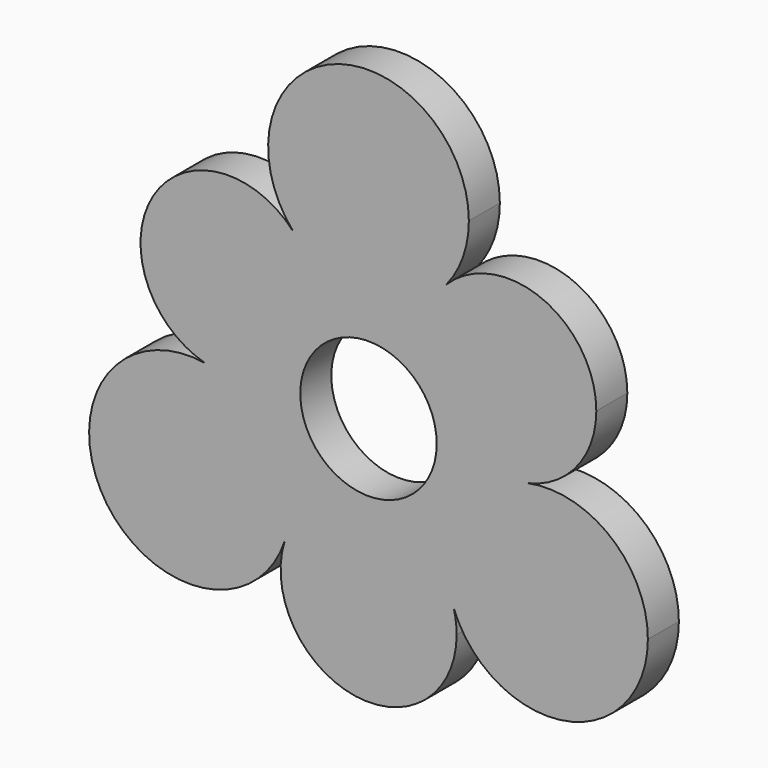
from build123d import *

# Parameters (mm, degrees)
F0_R     = 11.176
F1_DEPTH = 6.35


with BuildPart() as f1:
    # F0 (on Front) → F1 (new body)
    with BuildSketch(Plane.XZ):
        with BuildLine():
            ThreePointArc((12.7517006508, 23.4892014836), (15.490274076, 28.359134381), (16.4396849361, 33.8650085032))
            ThreePointArc((16.4396849361, 33.8650085032), (-5.7959286408, 49.2491058764), (-12.3528926478, 23.0174611293))
            ThreePointArc((-12.3528926478, 23.0174611293), (-12.2109180853, 22.8621908621), (-12.0712241226, 22.7048656287))
            ThreePointArc((-12.0712241226, 22.7048656287), (-0.3017671927, 17.4280934228), (11.6534468913, 22.2693016964))
            ThreePointArc((11.6534468913, 22.2693016964), (12.1852012792, 22.8948917308), (12.7517006508, 23.4892014836))
        make_face()
        with BuildLine():
            ThreePointArc((-12.0712241226, 22.7048656287), (-12.2109180853, 22.8621908621), (-12.3528926478, 23.0174611293))
            ThreePointArc((-12.3528926478, 23.0174611293), (-12.2130585437, 22.8602621723), (-12.0712241226, 22.7048656287))
        make_face()
        with BuildLine():
            ThreePointArc((-12.0712241226, 22.7048656287), (-12.2130585437, 22.8602621723), (-12.3528926478, 23.0174611293))
            ThreePointArc((-12.3528926478, 23.0174611293), (-35.2568762282, 20.6796890684), (-26.7180955248, -0.7013040367))
            ThreePointArc((-26.7180955248, -0.7013040367), (-25.9110393194, -0.8518354275), (-25.1125044392, -1.0424697987))
            ThreePointArc((-25.1125044392, -1.0424697987), (-13.5329586121, 2.2669935247), (-8.5036933239, 13.2097957122))
            ThreePointArc((-8.5036933239, 13.2097957122), (-9.4250093039, 18.2813740839), (-12.0712241226, 22.7048656287))
        make_face()
        with BuildLine():
            ThreePointArc((37.321032921, 13.2471223209), (28.4497702153, 26.5564449349), (12.7517006508, 23.4892014836))
            ThreePointArc((12.7517006508, 23.4892014836), (12.2178085396, 22.8655360028), (11.6534468913, 22.2693016964))
            ThreePointArc((11.6534468913, 22.2693016964), (10.5710761807, 5.7719047545), (25.6986024853, -0.8984460694))
            ThreePointArc((25.6986024853, -0.8984460694), (25.9040970502, -0.8533121295), (26.1101523925, -0.8108117214))
            ThreePointArc((26.1101523925, -0.8108117214), (34.1751435518, 4.2567197748), (37.321032921, 13.2471223209))
        make_face()
        with BuildLine():
            ThreePointArc((11.6534468913, 22.2693016964), (12.2178085396, 22.8655360028), (12.7517006508, 23.4892014836))
            ThreePointArc((12.7517006508, 23.4892014836), (12.1852012792, 22.8948917308), (11.6534468913, 22.2693016964))
        make_face()
        with BuildLine():
            ThreePointArc((-25.1125044392, -1.0424697987), (-25.9201584954, -0.8947520073), (-26.7180955248, -0.7013040367))
            ThreePointArc((-26.7180955248, -0.7013040367), (-43.4081977491, -25.41837957), (-13.7572597447, -22.2066494078))
            ThreePointArc((-13.7572597447, -22.2066494078), (-13.6937790301, -22.0060606965), (-13.6273783627, -21.8064195594))
            ThreePointArc((-13.6273783627, -21.8064195594), (-13.0740993856, -19.3973230871), (-12.8882727271, -16.9325042516))
            ThreePointArc((-12.8882727271, -16.9325042516), (-16.2979161501, -6.9084701851), (-25.1125044392, -1.0424697987))
        make_face()
        with BuildLine():
            ThreePointArc((-25.1125044392, -1.0424697987), (-25.9110393194, -0.8518354275), (-26.7180955248, -0.7013040367))
            ThreePointArc((-26.7180955248, -0.7013040367), (-25.9201584954, -0.8947520073), (-25.1125044392, -1.0424697987))
        make_face()
        with BuildLine():
            ThreePointArc((-13.6273783627, -21.8064195594), (-13.6937790301, -22.0060606965), (-13.7572597447, -22.2066494078))
            ThreePointArc((-13.7572597447, -22.2066494078), (-13.6910385066, -22.0069500429), (-13.6273783627, -21.8064195594))
        make_face()
        with BuildLine():
            ThreePointArc((-13.6273783627, -21.8064195594), (-13.6910385066, -22.0069500429), (-13.7572597447, -22.2066494078))
            ThreePointArc((-13.7572597447, -22.2066494078), (-2.127588621, -40.7153049273), (14.44099559, -26.4569180331))
            ThreePointArc((14.44099559, -26.4569180331), (14.3218531968, -24.6071235917), (13.966394874, -22.7878974469))
            ThreePointArc((13.966394874, -22.7878974469), (13.6932307798, -22.0137005753), (13.459057548, -21.2268318977))
            ThreePointArc((13.459057548, -21.2268318977), (-0.2869219447, -12.0407728951), (-13.6273783627, -21.8064195594))
        make_face()
        with BuildLine():
            ThreePointArc((26.1101523925, -0.8108117214), (25.9046971154, -0.8561301656), (25.6986024853, -0.8984460694))
            ThreePointArc((25.6986024853, -0.8984460694), (15.24405524, -8.4527086566), (13.459057548, -21.2268318977))
            ThreePointArc((13.459057548, -21.2268318977), (13.7349572161, -22.0001397234), (13.966394874, -22.7878974469))
            ThreePointArc((13.966394874, -22.7878974469), (32.3048678413, -33.100412174), (45.7676425992, -16.9325042516))
            ThreePointArc((45.7676425992, -16.9325042516), (39.7530124822, -4.2210341235), (26.1101523925, -0.8108117214))
        make_face()
        with BuildLine():
            ThreePointArc((26.1101523925, -0.8108117214), (25.9040970502, -0.8533121295), (25.6986024853, -0.8984460694))
            ThreePointArc((25.6986024853, -0.8984460694), (25.9046971154, -0.8561301656), (26.1101523925, -0.8108117214))
        make_face()
        with BuildLine():
            ThreePointArc((13.966394874, -22.7878974469), (13.7349572161, -22.0001397234), (13.459057548, -21.2268318977))
            ThreePointArc((13.459057548, -21.2268318977), (13.6932307798, -22.0137005753), (13.966394874, -22.7878974469))
        make_face()
        with BuildLine():
            ThreePointArc((11.6534468913, 22.2693016964), (-0.3017671927, 17.4280934228), (-12.0712241226, 22.7048656287))
            ThreePointArc((-12.0712241226, 22.7048656287), (-9.4250093039, 18.2813740839), (-8.5036933239, 13.2097957122))
            ThreePointArc((-8.5036933239, 13.2097957122), (-13.5329586121, 2.2669935247), (-25.1125044392, -1.0424697987))
            ThreePointArc((-25.1125044392, -1.0424697987), (-16.2979161501, -6.9084701851), (-12.8882727271, -16.9325042516))
            ThreePointArc((-12.8882727271, -16.9325042516), (-13.0740993856, -19.3973230871), (-13.6273783627, -21.8064195594))
            ThreePointArc((-13.6273783627, -21.8064195594), (-0.2869219447, -12.0407728951), (13.459057548, -21.2268318977))
            ThreePointArc((13.459057548, -21.2268318977), (15.24405524, -8.4527086566), (25.6986024853, -0.8984460694))
            ThreePointArc((25.6986024853, -0.8984460694), (10.5710761807, 5.7719047545), (11.6534468913, 22.2693016964))
        make_face()
        Circle(F0_R, mode=Mode.SUBTRACT)
    extrude(amount=F1_DEPTH)


solid = f1.part
